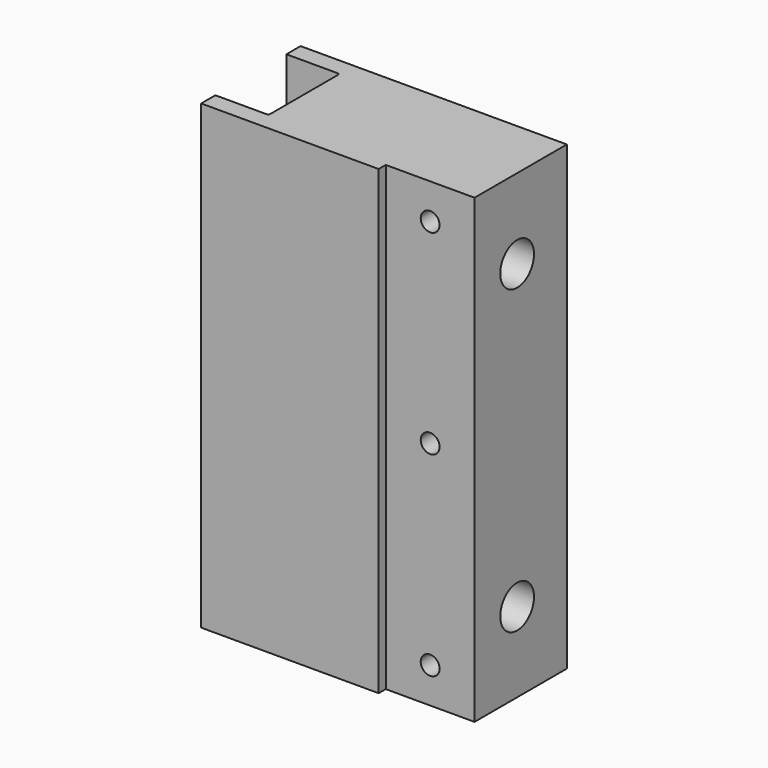
from build123d import *

# Parameters (mm, degrees)
F1_DEPTH       = 165.1
F2_R           = 1.524
F4_D           = 20.6375
F4_CBORE_D     = 30.1752
F4_CBORE_DEPTH = 28.448
F5_W           = 63.5
F5_H           = 330.2
F6_DEPTH       = 6.35
F8_D           = 13.49248
F8_DEPTH       = 41.2172727273
F8_TIP         = 4.0535499425


# Not quite as in the source:
# - a length typed as a fraction of an inch, garbled in the dataset ("3 / 203.2 mm" for 3/8 in), is restored


with BuildPart() as f1:
    # F0 (on Top) → F1 (new body, symmetric)
    with BuildSketch(Plane.XY):
        Polygon((95.25, 44.45), (-95.25, 44.45), (-95.25, 31.75), (-57.15, 31.75), (-57.15, -31.75), (-95.25, -31.75), (-95.25, -44.45), (95.25, -44.45), align=None)
    extrude(amount=F1_DEPTH, both=True)

    # F2
    f2_edges = [f1.edges().sort_by_distance(p)[0] for p in [
        (-57.15, 31.75, 0),
        (-57.15, -31.75, 0),
    ]]
    fillet(f2_edges, radius=F2_R)

    # F4 (through all)
    with Locations(Plane.YZ.offset(95.25)):
        with Locations((0, 107.95), (0, -107.95)):
            CounterBoreHole(F4_D / 2, F4_CBORE_D / 2, F4_CBORE_DEPTH)

    # F5 (on face) → F6 (cut)
    with BuildSketch(Plane.XZ.offset(44.45)):
        with Locations((63.5, 0)):
            Rectangle(F5_W, F5_H)
    extrude(amount=-F6_DEPTH, mode=Mode.SUBTRACT)

    # F8
    with Locations(Plane.XZ.offset(38.1)):
        with Locations((63.5, 139.7), (63.5, 0), (63.5, -139.7)):
            Hole(F8_D / 2, depth=F8_DEPTH)
            with Locations((0, 0, -(F8_DEPTH + F8_TIP / 2))):  # 118° drill point
                Cone(0, F8_D / 2, F8_TIP, mode=Mode.SUBTRACT)


solid = f1.part
